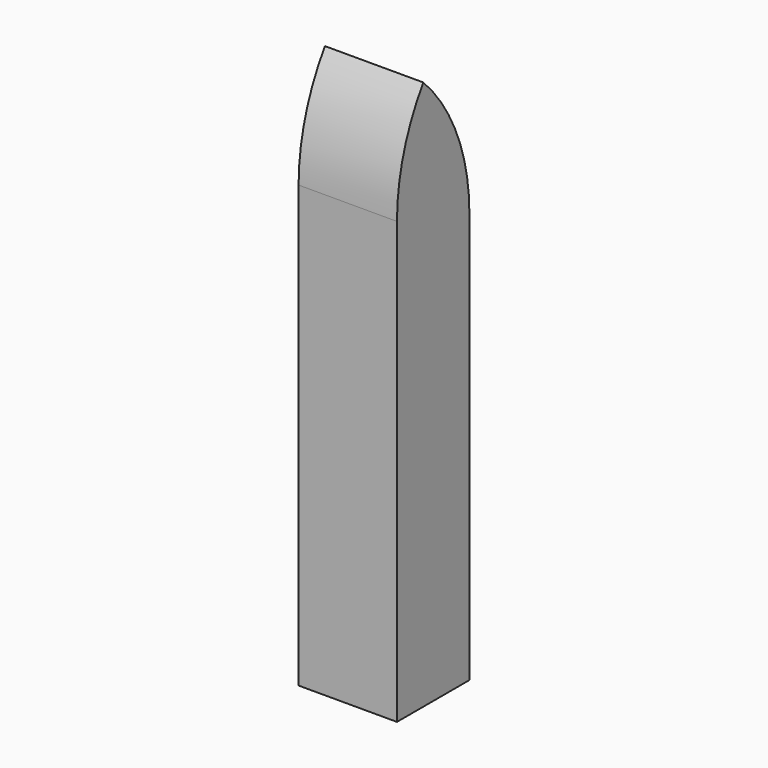
from build123d import *

# Parameters (mm, degrees)
F0_W        = 2.54
F0_H        = 2.3375834556
F1_DEPTH    = 25.4
F2_T1_DEPTH = 67.8607478943
F3_R        = 5.08
F4_T1_DEPTH = 20.8515396399


# Not quite as in the source:
# - a fillet or chamfer that OpenCascade refuses, or shapes differently, is made with other operations: its cross-section is extruded or revolved along the edge and cut away or added


with BuildPart() as f1:
    # F0 (on Top) → F1 (new body)
    with BuildSketch(Plane.XY):
        with Locations((13.1794903427, -0.4677381366)):
            Rectangle(F0_W, F0_H)
    extrude(amount=F1_DEPTH)

    # F2: chamfer of 12.7 on 1 edges, made by hand

    # F2_s2 → F2_t1 (cut)
    with BuildSketch(Plane.YZ.offset(-20.7508836044)):
        Polygon((0.7010535912, 12.7), (-11.9989464088, 25.4), (0.7010535912, 25.4), align=None)
    extrude(amount=F2_T1_DEPTH, mode=Mode.SUBTRACT)

    # F3
    f3_edges = [f1.edges().sort_by_distance(p)[0] for p in [
        (13.17949, 0.701054, 12.7),
    ]]
    fillet(f3_edges, radius=F3_R)

    # F4: fillet of radius 5.08 on 1 edges, made by hand

    # F4_s2 → F4_t1 (cut)
    with BuildSketch(Plane.YZ.offset(2.7537205228)):
        with BuildLine():
            ThreePointArc((-0.7868439604, 14.1878975516), (-1.4194711353, 12.8443576208), (-1.6365298645, 11.3752755277))
            Line((-1.6365298645, 11.3752755277), (-1.6365298645, 15.0375834557))
            Line((-1.6365298645, 15.0375834557), (-0.7868439604, 14.1878975516))
        make_face()
    extrude(amount=F4_T1_DEPTH, mode=Mode.SUBTRACT)


solid = f1.part
